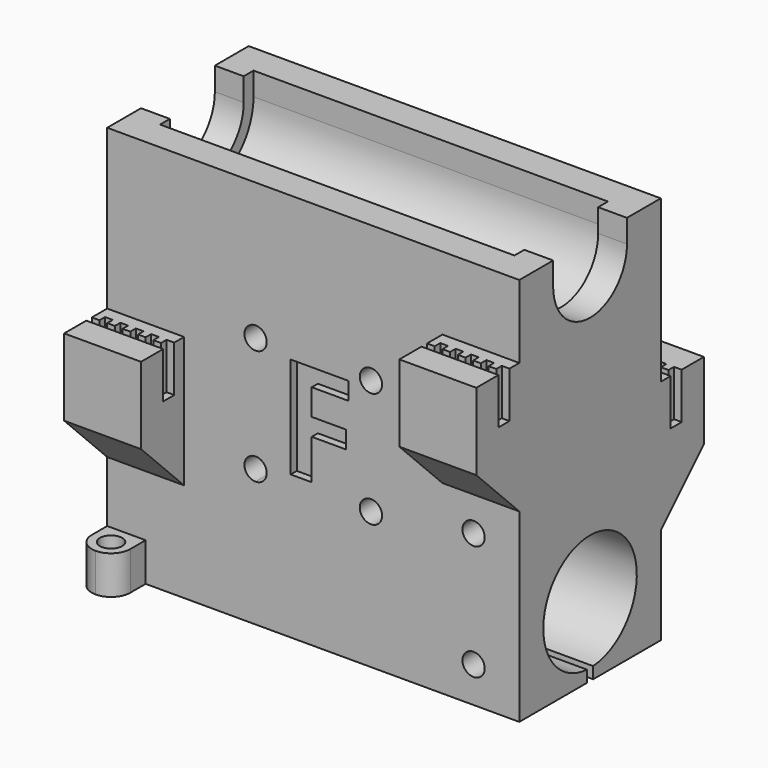
from build123d import *

# Parameters (mm, degrees)
F1_W          = 53.6
F1_H          = 23
F2_DEPTH      = 50.6
F4_DEPTH      = 53.601
F5_DEPTH      = 49.85
F6_DEPTH      = 24.95
F7_DEPTH      = 25.05
F8_DEPTH      = 3.75
F9_W          = 10
F9_H          = 20
F10_DEPTH     = 7
F11_T4_DEPTH  = 61.4336597593
F11_T9_DEPTH  = 61.4336597593
F13_DEPTH     = 6
F15_DEPTH     = 6
F16_W         = 10
F16_H         = 20
F17_DEPTH     = 7
F19_DEPTH     = 6
F21_DEPTH     = 6
F22_T4_DEPTH  = 61.4336597593
F22_T9_DEPTH  = 61.4336597593
F23_R         = 1.45
F24_DEPTH     = 30.001
F25_R         = 1.45
F26_DEPTH     = 5
F27_TEXT_SIZE = 18.4411155982
F28_DEPTH     = 1
F29_W         = 5
F29_H         = 5
F30_DEPTH     = 5
F31_R         = 1.45
F32_DEPTH     = 25
F33_R         = 2.49999


# Not quite as in the source:
# - a fillet or chamfer that OpenCascade refuses, or shapes differently, is made with other operations: its cross-section is extruded or revolved along the edge and cut away or added
# - a fillet or chamfer is up to 0.001 mm smaller than in the source, because OpenCascade refuses the exact size
# - a feature names something its author has since deleted; it is built from what else it names
# - Text() gives the source's letters only with a copy of the font that has no kerning and outlines rounded to 1/6400 em; it was checked with that copy


with BuildPart() as f2:
    # F1 (on Top) → F2 (new body)
    with BuildSketch(Plane.XY):
        with Locations((26.8, 11.5)):
            Rectangle(F1_W, F1_H)
    extrude(amount=F2_DEPTH)

    # F3 (on face) → F4 (cut, through all)
    with BuildSketch(Plane(origin=(0, 0, 0), x_dir=(0, -1, 0), z_dir=(-1, 0, 0))):
        with BuildLine():
            ThreePointArc((-11, 1.5164652041), (-11.5, 1.5), (-12, 1.5164652041))
            Line((-12, 1.5164652041), (-12, 0))
            Line((-12, 0), (-11.5, 0))
            Line((-11.5, 0), (-11, 0))
            Line((-11, 0), (-11, 1.5164652041))
        make_face()
        with BuildLine():
            Line((-11, 1.5164652041), (-12, 1.5164652041))
            ThreePointArc((-12, 1.5164652041), (-11.5, 1.5), (-11, 1.5164652041))
        make_face()
        with BuildLine():
            ThreePointArc((-11, 1.5164652041), (-5.9520273973, 3.9057724347), (-3.9, 9.1))
            ThreePointArc((-3.9, 9.1), (-16.6942275653, 14.6479726027), (-12, 1.5164652041))
            Line((-12, 1.5164652041), (-11, 1.5164652041))
        make_face()
        with BuildLine():
            Line((-5.5, 47.6), (-5.5, 50.6))
            Line((-5.5, 50.6), (-6.3038475773, 50.6))
            ThreePointArc((-6.3038475773, 50.6), (-5.7044450423, 49.1529142706), (-5.5, 47.6))
        make_face()
        with BuildLine():
            Line((-16.6961524227, 50.6), (-17.5, 50.6))
            Line((-17.5, 50.6), (-17.5, 47.6))
            ThreePointArc((-17.5, 47.6), (-17.2955549577, 49.1529142706), (-16.6961524227, 50.6))
        make_face()
        with BuildLine():
            ThreePointArc((-16.6961524227, 50.6), (-17.2955549577, 49.1529142706), (-17.5, 47.6))
            ThreePointArc((-17.5, 47.6), (-11.5, 41.6), (-5.5, 47.6))
            ThreePointArc((-5.5, 47.6), (-5.7044450423, 49.1529142706), (-6.3038475773, 50.6))
            Line((-6.3038475773, 50.6), (-16.6961524227, 50.6))
        make_face()
    extrude(amount=-F4_DEPTH, mode=Mode.SUBTRACT)

    # F3 (on face) → F5 (cut)
    with BuildSketch(Plane(origin=(0, 0, 0), x_dir=(0, -1, 0), z_dir=(-1, 0, 0))):
        with BuildLine():
            ThreePointArc((-18.4828361, 50.6), (-18.9441102343, 49.1314120346), (-19.1, 47.6))
            ThreePointArc((-19.1, 47.6), (-11.5, 40), (-3.9, 47.6))
            ThreePointArc((-3.9, 47.6), (-4.0558897657, 49.1314120346), (-4.5171639, 50.6))
            Line((-4.5171639, 50.6), (-5.5, 50.6))
            Line((-5.5, 50.6), (-5.5, 47.6))
            ThreePointArc((-5.5, 47.6), (-11.5, 41.6), (-17.5, 47.6))
            Line((-17.5, 47.6), (-17.5, 50.6))
            Line((-17.5, 50.6), (-18.4828361, 50.6))
        make_face()
        with BuildLine():
            Line((-18.4828361, 50.6), (-19.1, 50.6))
            Line((-19.1, 50.6), (-19.1, 47.6))
            ThreePointArc((-19.1, 47.6), (-18.9441102343, 49.1314120346), (-18.4828361, 50.6))
        make_face()
        with BuildLine():
            Line((-3.9, 47.6), (-3.9, 50.6))
            Line((-3.9, 50.6), (-4.5171639, 50.6))
            ThreePointArc((-4.5171639, 50.6), (-4.0558897657, 49.1314120346), (-3.9, 47.6))
        make_face()
    extrude(amount=-F5_DEPTH, mode=Mode.SUBTRACT)

    # F3 (on face) → F6 (join)
    with BuildSketch(Plane(origin=(0, 0, 0), x_dir=(0, -1, 0), z_dir=(-1, 0, 0))):
        with BuildLine():
            ThreePointArc((-18.4828361, 50.6), (-18.9441102343, 49.1314120346), (-19.1, 47.6))
            ThreePointArc((-19.1, 47.6), (-11.5, 40), (-3.9, 47.6))
            ThreePointArc((-3.9, 47.6), (-4.0558897657, 49.1314120346), (-4.5171639, 50.6))
            Line((-4.5171639, 50.6), (-5.5, 50.6))
            Line((-5.5, 50.6), (-5.5, 47.6))
            ThreePointArc((-5.5, 47.6), (-11.5, 41.6), (-17.5, 47.6))
            Line((-17.5, 47.6), (-17.5, 50.6))
            Line((-17.5, 50.6), (-18.4828361, 50.6))
        make_face()
        with BuildLine():
            Line((-18.4828361, 50.6), (-19.1, 50.6))
            Line((-19.1, 50.6), (-19.1, 47.6))
            ThreePointArc((-19.1, 47.6), (-18.9441102343, 49.1314120346), (-18.4828361, 50.6))
        make_face()
        with BuildLine():
            Line((-3.9, 47.6), (-3.9, 50.6))
            Line((-3.9, 50.6), (-4.5171639, 50.6))
            ThreePointArc((-4.5171639, 50.6), (-4.0558897657, 49.1314120346), (-3.9, 47.6))
        make_face()
    extrude(amount=-F6_DEPTH)

    # F3 (on face) → F7 (cut)
    with BuildSketch(Plane(origin=(0, 0, 0), x_dir=(0, -1, 0), z_dir=(-1, 0, 0))):
        with BuildLine():
            ThreePointArc((-18.4828361, 50.6), (-18.9441102343, 49.1314120346), (-19.1, 47.6))
            ThreePointArc((-19.1, 47.6), (-11.5, 40), (-3.9, 47.6))
            ThreePointArc((-3.9, 47.6), (-4.0558897657, 49.1314120346), (-4.5171639, 50.6))
            Line((-4.5171639, 50.6), (-5.5, 50.6))
            Line((-5.5, 50.6), (-5.5, 47.6))
            ThreePointArc((-5.5, 47.6), (-11.5, 41.6), (-17.5, 47.6))
            Line((-17.5, 47.6), (-17.5, 50.6))
            Line((-17.5, 50.6), (-18.4828361, 50.6))
        make_face()
        with BuildLine():
            Line((-18.4828361, 50.6), (-19.1, 50.6))
            Line((-19.1, 50.6), (-19.1, 47.6))
            ThreePointArc((-19.1, 47.6), (-18.9441102343, 49.1314120346), (-18.4828361, 50.6))
        make_face()
        with BuildLine():
            Line((-3.9, 47.6), (-3.9, 50.6))
            Line((-3.9, 50.6), (-4.5171639, 50.6))
            ThreePointArc((-4.5171639, 50.6), (-4.0558897657, 49.1314120346), (-3.9, 47.6))
        make_face()
    extrude(amount=-F7_DEPTH, mode=Mode.SUBTRACT)

    # F3 (on face) → F8 (join)
    with BuildSketch(Plane(origin=(0, 0, 0), x_dir=(0, -1, 0), z_dir=(-1, 0, 0))):
        with BuildLine():
            ThreePointArc((-18.4828361, 50.6), (-18.9441102343, 49.1314120346), (-19.1, 47.6))
            ThreePointArc((-19.1, 47.6), (-11.5, 40), (-3.9, 47.6))
            ThreePointArc((-3.9, 47.6), (-4.0558897657, 49.1314120346), (-4.5171639, 50.6))
            Line((-4.5171639, 50.6), (-5.5, 50.6))
            Line((-5.5, 50.6), (-5.5, 47.6))
            ThreePointArc((-5.5, 47.6), (-11.5, 41.6), (-17.5, 47.6))
            Line((-17.5, 47.6), (-17.5, 50.6))
            Line((-17.5, 50.6), (-18.4828361, 50.6))
        make_face()
        with BuildLine():
            Line((-18.4828361, 50.6), (-19.1, 50.6))
            Line((-19.1, 50.6), (-19.1, 47.6))
            ThreePointArc((-19.1, 47.6), (-18.9441102343, 49.1314120346), (-18.4828361, 50.6))
        make_face()
        with BuildLine():
            Line((-3.9, 47.6), (-3.9, 50.6))
            Line((-3.9, 50.6), (-4.5171639, 50.6))
            ThreePointArc((-4.5171639, 50.6), (-4.0558897657, 49.1314120346), (-3.9, 47.6))
        make_face()
    extrude(amount=-F8_DEPTH)

    # F9 (on face) → F10 (join)
    with BuildSketch(Plane.XZ):
        with Locations((5, 19.9)):
            Rectangle(F9_W, F9_H)
        with Locations((48.6, 31.1)):
            Rectangle(F9_W, F9_H)
    extrude(amount=F10_DEPTH)

    # F11: chamfer of 10 on 2 edges, made by hand


with BuildPart() as f11_tool2:
    # F11_s3 → F11_t4 (new body)
    with BuildSketch(Plane.YZ.offset(-25.7168298797)):
        Polygon((3, 9.9), (-7, 19.9), (-7, 9.9), align=None)
    extrude(amount=F11_T4_DEPTH)

    split(bisect_by=Plane.XZ, keep=Keep.TOP)


with BuildPart() as f2_1:
    add(f2.part)

    # F11_t1: cut F11_tool2
    add(f11_tool2.part, mode=Mode.SUBTRACT)


with BuildPart() as f11_tool7:
    # F11_s8 → F11_t9 (new body)
    with BuildSketch(Plane.YZ.offset(17.8831701203)):
        Polygon((3, 21.1), (-7, 31.1), (-7, 21.1), align=None)
    extrude(amount=F11_T9_DEPTH)

    split(bisect_by=Plane.XZ, keep=Keep.TOP)


with BuildPart() as f2_2:
    add(f2_1.part)

    # F11_t6: cut F11_tool7
    add(f11_tool7.part, mode=Mode.SUBTRACT)

    # F12 (on face) → F13 (cut)
    with BuildSketch(Plane.XY.offset(29.9)):
        Polygon((0, -2.5), (0, -3.4), (10, -3.4), (10, -2.5), (10, -1.6), (9, -1.6), (9, -2.5), (8, -2.5), (8, -1.6), (7, -1.6), (7, -2.5), (6, -2.5), (6, -1.6), (5.2958247252, -1.6), (5, -1.6), (5, -2.5), (4, -2.5), (4, -1.6), (3, -1.6), (3, -2.5), (2, -2.5), (2, -1.6), (1, -1.6), (1, -2.5), align=None)
    extrude(amount=-F13_DEPTH, mode=Mode.SUBTRACT)

    # F14 (on face) → F15 (cut)
    with BuildSketch(Plane.XY.offset(41.1)):
        Polygon((43.6, -2.5), (43.6, -3.4), (53.6, -3.4), (53.6, -2.5), (53.6, -1.6), (52.6, -1.6), (52.6, -2.5), (51.6, -2.5), (51.6, -1.6), (50.6, -1.6), (50.6, -2.5), (49.6, -2.5), (49.6, -1.6), (48.8349036932, -1.6), (48.6, -1.6), (48.6, -2.5), (47.6, -2.5), (47.6, -1.6), (46.6, -1.6), (46.6, -2.5), (45.6, -2.5), (45.6, -1.6), (44.6, -1.6), (44.6, -2.5), align=None)
    extrude(amount=-F15_DEPTH, mode=Mode.SUBTRACT)

    # F16 (on face) → F17 (join)
    with BuildSketch(Plane(origin=(0, 23, 0), x_dir=(-1, 0, 0), z_dir=(0, 1, 0))):
        with Locations((-48.6, 19.6)):
            Rectangle(F16_W, F16_H)
        with Locations((-5, 31.1)):
            Rectangle(F16_W, F16_H)
    extrude(amount=F17_DEPTH)

    # F18 (on face) → F19 (cut)
    with BuildSketch(Plane.XY.offset(29.6)):
        Polygon((43.6, 25.5), (43.6, 24.6), (48.6, 24.6), (53.6, 24.6), (53.6, 25.5), (53.6, 26.4), (52.6, 26.4), (52.6, 25.5), (51.6, 25.5), (51.6, 26.4), (50.6, 26.4), (50.6, 25.5), (49.6, 25.5), (49.6, 26.4), (48.6, 26.4), (48.6, 25.5), (47.6, 25.5), (47.6, 26.4), (46.6, 26.4), (46.6, 25.5), (45.6, 25.5), (45.6, 26.4), (44.6, 26.4), (44.6, 25.5), align=None)
    extrude(amount=-F19_DEPTH, mode=Mode.SUBTRACT)

    # F20 (on face) → F21 (cut)
    with BuildSketch(Plane.XY.offset(41.1)):
        Polygon((7, 25.5), (6, 25.5), (6, 26.4), (5, 26.4), (5, 25.5), (4, 25.5), (4, 26.4), (3, 26.4), (3, 25.5), (2, 25.5), (2, 26.4), (1, 26.4), (1, 25.5), (0, 25.5), (0, 24.6), (5, 24.6), (10, 24.6), (10, 25.5), (10, 26.4), (9, 26.4), (9, 25.5), (8, 25.5), (8, 26.4), (7, 26.4), align=None)
    extrude(amount=-F21_DEPTH, mode=Mode.SUBTRACT)

    # F22: chamfer of 10 on 2 edges, made by hand


with BuildPart() as f22_tool2:
    # F22_s3 → F22_t4 (new body)
    with BuildSketch(Plane.YZ.offset(35.7168298797)):
        Polygon((30, 31.1), (20, 21.1), (30, 21.1), align=None)
    extrude(amount=-F22_T4_DEPTH)

    split(bisect_by=Plane.XZ.offset(-23), keep=Keep.BOTTOM)


with BuildPart() as f2_3:
    add(f2_2.part)

    # F22_t1: cut F22_tool2
    add(f22_tool2.part, mode=Mode.SUBTRACT)


with BuildPart() as f22_tool7:
    # F22_s8 → F22_t9 (new body)
    with BuildSketch(Plane.YZ.offset(79.3168298797)):
        Polygon((20, 9.6), (30, 19.6), (30, 9.6), align=None)
    extrude(amount=-F22_T9_DEPTH)

    split(bisect_by=Plane.XZ.offset(-23), keep=Keep.BOTTOM)


with BuildPart() as f2_4:
    add(f2_3.part)

    # F22_t6: cut F22_tool7
    add(f22_tool7.part, mode=Mode.SUBTRACT)

    # F23 (on face) → F24 (cut, through all)
    with BuildSketch(Plane.XZ):
        with BuildLine():
            ThreePointArc((17.85, 32.8), (19.3, 31.35), (20.75, 32.8))
            ThreePointArc((20.75, 32.8), (19.3, 34.25), (17.85, 32.8))
        make_face()
        with BuildLine():
            ThreePointArc((35.75, 32.8), (35.3253048327, 33.8253048327), (34.3, 34.25))
            ThreePointArc((34.3, 34.25), (33.2746951673, 31.7746951673), (35.75, 32.8))
        make_face()
        with BuildLine():
            ThreePointArc((20.75, 17.8), (18.2746951673, 18.8253048327), (19.3, 16.35))
            ThreePointArc((19.3, 16.35), (20.3253048327, 16.7746951673), (20.75, 17.8))
        make_face()
        with Locations((34.3, 17.8)):
            Circle(F23_R)
    extrude(amount=-F24_DEPTH, mode=Mode.SUBTRACT)

    # F25 (on face) → F26 (cut)
    with BuildSketch(Plane.XZ):
        with Locations((47.65, 19.65)):
            Circle(F25_R)
        with Locations((47.65, 4.65)):
            Circle(F25_R)
    extrude(amount=-F26_DEPTH, mode=Mode.SUBTRACT)

    # F27 (on face) → F28 (cut)
    with BuildSketch(Plane.XZ):
        with Locations((22.1983653734, 18.6611983846)):
            Text('F', F27_TEXT_SIZE, font='Open Sans', font_style=FontStyle.BOLD, text_align=(TextAlign.LEFT, TextAlign.BOTTOM))
    extrude(amount=-F28_DEPTH, mode=Mode.SUBTRACT)

    # F29 (on face) → F30 (join)
    with BuildSketch(Plane.XZ):
        with Locations((2.5, 2.5)):
            Rectangle(F29_W, F29_H)
    extrude(amount=F30_DEPTH)

    # F31 (on face) → F32 (cut)
    with BuildSketch(Plane.XY.offset(5)):
        with Locations((2.5, -2.5)):
            Circle(F31_R)
    extrude(amount=-F32_DEPTH, mode=Mode.SUBTRACT)

    # F33 (radius 2.5 in the source; OpenCascade refuses exactly that, so slightly less here)
    f33_edges = [f2_4.edges().sort_by_distance(p)[0] for p in [
        (0, -5, 2.5),
        (5, -5, 2.5),
    ]]
    fillet(f33_edges, radius=F33_R)


solid = f2_4.part
